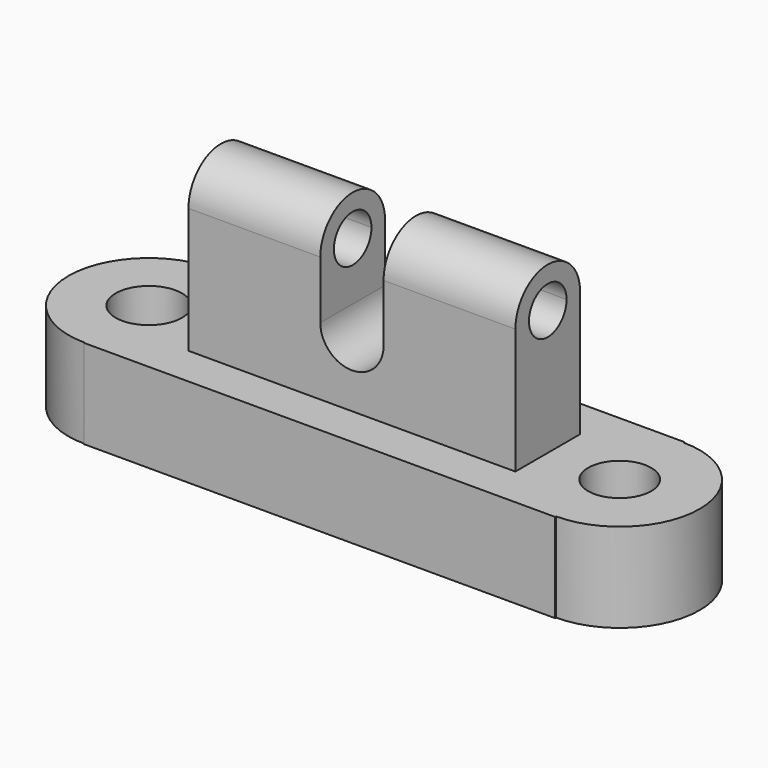
from build123d import *

# Parameters (mm, degrees)
F2_DEPTH      = 13.8532817364
F1_R          = 5.1568283111
F1_R_2        = 4.9060467952
F3_DEPTH      = 19.6482334286
F4_DEPTH      = 33.8999927044
F6_DEPTH      = 25.4
F6_DEPTH_BACK = 25.4
F8_DEPTH      = 25.4
F8_DEPTH_BACK = 25.4


with BuildPart() as f2:
    # F0 (on Top) → F2 (new body)
    with BuildSketch(Plane.XY):
        with BuildLine():
            Line((36.6003066301, 12.4013655132), (36.6003066301, 12.5824138522))
            Line((36.6003066301, 12.5824138522), (-36.6003066301, 12.5824138522))
            Line((-36.6003066301, 12.5824138522), (-36.6003066301, 12.4739914422))
            ThreePointArc((-36.6003066301, 12.4739914422), (-49.0742980723, 0), (-36.6003066301, -12.4739914422))
            Line((-36.6003066301, -12.4739914422), (-36.6003066301, -12.5824138522))
            Line((-36.6003066301, -12.5824138522), (36.6003066301, -12.5824138522))
            Line((36.6003066301, -12.5824138522), (36.6003066301, -12.4013655132))
            ThreePointArc((36.6003066301, -12.4013655132), (49.0016721433, 0), (36.6003066301, 12.4013655132))
        make_face()
    extrude(amount=F2_DEPTH)


with BuildPart() as f2b:
    # F1 (on Top) → F2, piece 2 (new body)
    with BuildSketch(Plane.XY):
        with Locations((-36.5818925202, 0)):
            Circle(F1_R)
    extrude(amount=F2_DEPTH)


with BuildPart() as f2c:
    # F1 (on Top) → F2, piece 3 (new body)
    with BuildSketch(Plane.XY):
        with Locations((36.5750528872, 0)):
            Circle(F1_R_2)
    extrude(amount=F2_DEPTH)


with BuildPart() as f3_tool:
    # F3 (cut): a face of the model
    f3_faces = [f2c.part.faces().sort_by_distance(p)[0] for p in [
        (36.5750528872, 0, 13.8532817364),
    ]]
    extrude(f3_faces, amount=-F3_DEPTH)


with BuildPart() as f2_1:
    add(f2.part)

    # F3: cut by f3_tool
    add(f3_tool.part, mode=Mode.SUBTRACT)


with BuildPart() as f2c_1:
    add(f2c.part)

    # F3: cut by f3_tool
    add(f3_tool.part, mode=Mode.SUBTRACT)


with BuildPart() as f4_tool:
    # F4 (cut): a face of the model
    f4_faces = [f2b.part.faces().sort_by_distance(p)[0] for p in [
        (-36.5818925202, 0, 13.8532817364),
    ]]
    extrude(f4_faces, amount=-F4_DEPTH)


with BuildPart() as f2_2:
    add(f2_1.part)

    # F4: cut by f4_tool
    add(f4_tool.part, mode=Mode.SUBTRACT)

    # F5 (on Right) → F6 (join, two sides)
    with BuildSketch(Plane.YZ) as f6_sk:
        with BuildLine():
            ThreePointArc((-6.2862960622, 33.3382003009), (0, 27.0519042388), (6.2862960622, 33.3382003009))
            Line((6.2862960622, 33.3382003009), (3.6514560074, 33.3382003009))
            ThreePointArc((3.6514560074, 33.3382003009), (0, 29.6867442936), (-3.6514560074, 33.3382003009))
            Line((-3.6514560074, 33.3382003009), (-6.2862960622, 33.3382003009))
        make_face()
        with BuildLine():
            Line((3.6514560074, 33.3382003009), (6.2862960622, 33.3382003009))
            ThreePointArc((6.2862960622, 33.3382003009), (0, 39.6244963631), (-6.2862960622, 33.3382003009))
            Line((-6.2862960622, 33.3382003009), (-3.6514560074, 33.3382003009))
            ThreePointArc((-3.6514560074, 33.3382003009), (0, 36.9896563083), (3.6514560074, 33.3382003009))
        make_face()
        with BuildLine():
            Line((6.2862960622, 4.7357268631), (6.2862960622, 33.3382003009))
            ThreePointArc((6.2862960622, 33.3382003009), (0, 27.0519042388), (-6.2862960622, 33.3382003009))
            Line((-6.2862960622, 33.3382003009), (-6.2862960622, 4.7357268631))
            Line((-6.2862960622, 4.7357268631), (6.2862960622, 4.7357268631))
        make_face()
    extrude(amount=F6_DEPTH)
    extrude(f6_sk.sketch, amount=-F6_DEPTH_BACK)

    # F7 (on Front) → F8 (cut, two sides)
    with BuildSketch(Plane.XZ) as f8_sk:
        with BuildLine():
            Line((4.9151992425, 24.3559591472), (4.9151992425, 50.461564213))
            Line((4.9151992425, 50.461564213), (-4.9151992425, 50.461564213))
            Line((-4.9151992425, 50.461564213), (-4.9151992425, 24.3559591472))
            ThreePointArc((-4.9151992425, 24.3559591472), (0, 29.2711583897), (4.9151992425, 24.3559591472))
        make_face()
        with BuildLine():
            ThreePointArc((-4.9151992425, 24.3559591472), (0, 19.4407599047), (4.9151992425, 24.3559591472))
            Line((4.9151992425, 24.3559591472), (-4.9151992425, 24.3559591472))
        make_face()
        with BuildLine():
            Line((-4.9151992425, 24.3559591472), (4.9151992425, 24.3559591472))
            ThreePointArc((4.9151992425, 24.3559591472), (0, 29.2711583897), (-4.9151992425, 24.3559591472))
        make_face()
    extrude(amount=-F8_DEPTH, mode=Mode.SUBTRACT)
    extrude(f8_sk.sketch, amount=F8_DEPTH_BACK, mode=Mode.SUBTRACT)


with BuildPart() as f2b_1:
    add(f2b.part)

    # F4: cut by f4_tool
    add(f4_tool.part, mode=Mode.SUBTRACT)


solid = f2_2.part
